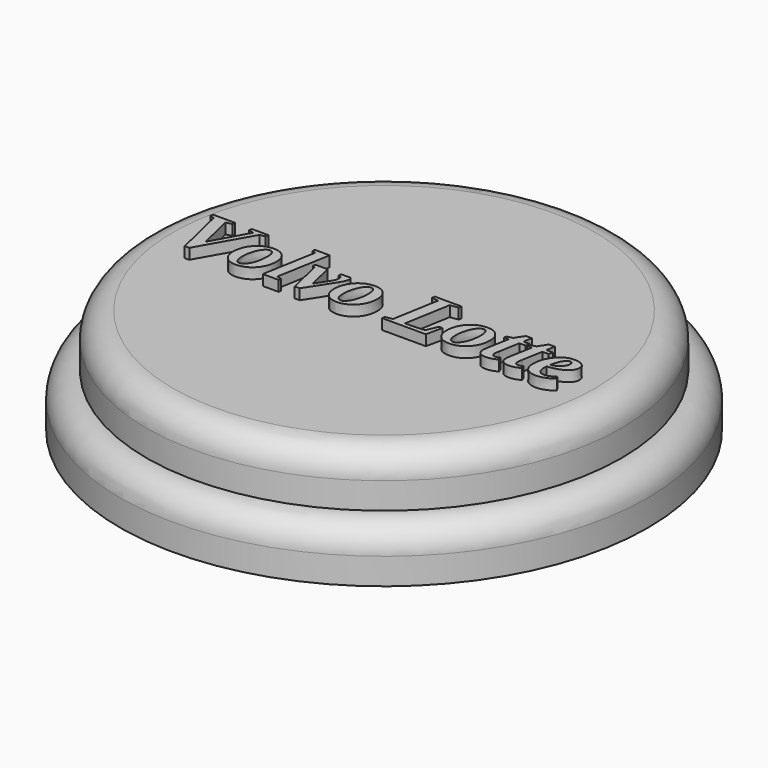
from build123d import *

# Parameters (mm, degrees)
F0_R         = 50
F1_DEPTH     = 10
F2_R         = 45
F3_DEPTH     = 10
F4_R         = 4.99999
F6_TEXT_SIZE = 15.6591524484
F7_DEPTH     = 2


# Not quite as in the source:
# - a fillet or chamfer is up to 0.001 mm smaller than in the source, because OpenCascade refuses the exact size
# - Text() gives the source's letters only with a copy of the font that has no kerning and outlines rounded to 1/6400 em; it was checked with that copy


with BuildPart() as f1:
    # F0 (on Top) → F1 (new body)
    with BuildSketch(Plane.XY):
        Circle(F0_R)
    extrude(amount=F1_DEPTH)

    # F2 (on face) → F3 (join)
    with BuildSketch(Plane.XY.offset(10)):
        Circle(F2_R)
    extrude(amount=F3_DEPTH)

    # F4 (radius 5 in the source; OpenCascade refuses exactly that, so slightly less here)
    f4_edges = [f1.edges().sort_by_distance(p)[0] for p in [
        (-50, 0, 10),
        (-45, 0, 20),
    ]]
    fillet(f4_edges, radius=F4_R)

    # F6 (on face) → F7 (join)
    with BuildSketch(Plane.XY.offset(20)):
        with Locations((-37.5, -5.1264656666)):
            Text('Volvo Lotte', F6_TEXT_SIZE, font='Tinos', font_style=FontStyle.BOLDITALIC, text_align=(TextAlign.LEFT, TextAlign.BOTTOM))
    extrude(amount=F7_DEPTH)


solid = f1.part
